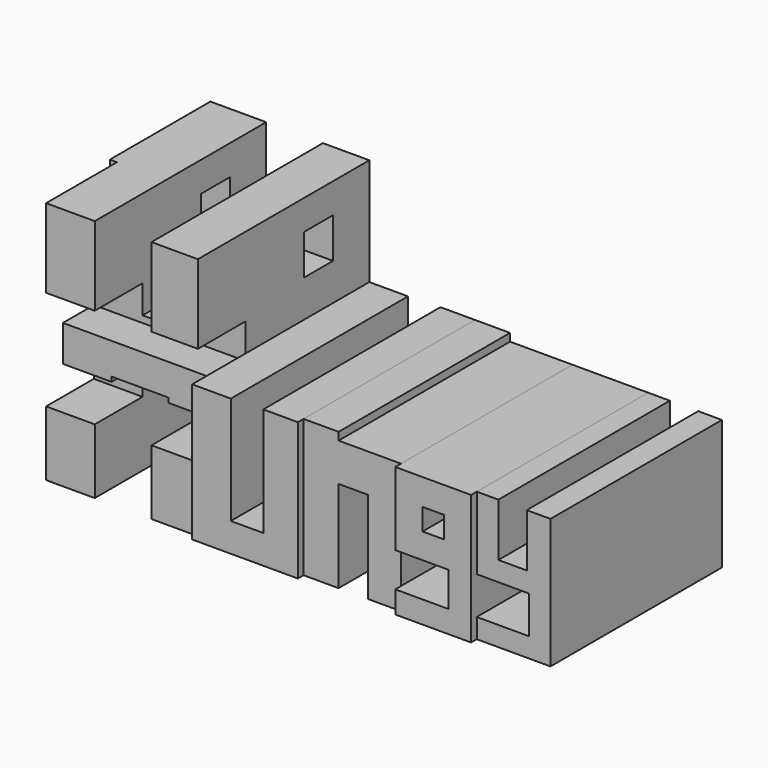
from build123d import *

# Parameters (mm, degrees)
F1_DEPTH = 76.2
F2_DEPTH = 78.74
F0_W     = 7.6985582709
F0_H     = 7.6985568739
F3_W     = 19.2463956773
F3_H     = 4.9490719102
F3_W_2   = 12.830927968
F3_H_2   = 14.2973195761
F3_H_3   = 10.814640671
F4_DEPTH = 179.3468610773
F5_DEPTH = 2.54


with BuildPart() as f1:
    # F0 (on Front) → F1 (new body)
    with BuildSketch(Plane.XZ):
        Polygon((-93.9285457134, 43.3502085507), (-93.9285457134, -43.3502085507), (-76.6189694405, -43.3502085507), (-76.6189694405, -8.3401026204), (-56.4560815692, -8.3401026204), (-56.4560815692, -43.3502085507), (-39.9591773748, -43.3502085507), (-39.9591773748, 5.224020686), (-39.9591773748, 43.3502085507), (-56.4560815692, 43.3502085507), (-56.4560815692, 5.224020686), (-76.6189694405, 5.224020686), (-76.6189694405, 43.3502085507), align=None)
    extrude(amount=F1_DEPTH)

    # F3 (on face) → F4 (cut, through all)
    with BuildSketch(Plane(origin=(-93.9285457134, 0, 0), x_dir=(0, -1, 0), z_dir=(-1, 0, 0))):
        with Locations((35.0886601955, -0.377497403)):
            Rectangle(F3_W, F3_H)
        Polygon((76.2, -20.2654339373), (76.2, 15.2945648879), (54.9766011536, 15.2945648879), (54.9766011536, 2.8302345891), (68.7240213156, 2.8302345891), (68.7240213156, -10.0006936118), (54.9766011536, -10.0006936118), (54.9766011536, -20.2654339373), align=None)
        with Locations((22.5326810032, 25.559307076)):
            Rectangle(F3_W_2, F3_H_2)
        with Locations((22.5326810032, -23.1065694243)):
            Rectangle(F3_W_2, F3_H_3)
    extrude(amount=-F4_DEPTH, mode=Mode.SUBTRACT)

    # F3 (on face) → F5 (join)
    with BuildSketch(Plane(origin=(-93.9285457134, 0, 0), x_dir=(0, -1, 0), z_dir=(-1, 0, 0))):
        Polygon((44.7118580341, 43.3502085507), (0, 43.3502085507), (0, -43.3502085507), (44.7118580341, -43.3502085507), (44.7118580341, -2.8520333581), (25.4654623568, -2.8520333581), (25.4654623568, 2.0970385522), (44.7118580341, 2.0970385522), align=None)
        with Locations((22.5326810032, -23.1065694243)):
            Rectangle(F3_W_2, F3_H_3, mode=Mode.SUBTRACT)
        with Locations((22.5326810032, 25.559307076)):
            Rectangle(F3_W_2, F3_H_2, mode=Mode.SUBTRACT)
    extrude(amount=F5_DEPTH)


with BuildPart() as f1b:
    # F0 (on Front) → F1, piece 2 (new body)
    with BuildSketch(Plane.XZ):
        Polygon((-2.3828870617, 5.590618588), (-2.3828870617, -43.3502085507), (10.081442073, -43.3502085507), (10.081442073, -10.7229892164), (20.529486239, -10.7229892164), (20.529486239, -43.3502085507), (32.2606191039, -43.3502085507), (32.2606191039, -35.4683510959), (32.2606191039, -23.1873188168), (32.2606191039, -10.7229892164), (32.2606191039, 2.8411338571), (10.081442073, 2.8411338571), (10.081442073, 5.590618588), align=None)
    extrude(amount=F1_DEPTH)


with BuildPart() as f1c:
    # F0 (on Front) → F1, piece 3 (new body)
    with BuildSketch(Plane.XZ):
        Polygon((66.9041201472, 2.8411338571), (59.2055656016, 2.8411338571), (59.2055656016, -23.0040214956), (77.7187645435, -23.0040214956), (77.7187645435, -36.3848470151), (59.2055656016, -36.3848470151), (59.2055656016, -43.3502085507), (77.7187645435, -43.3502085507), (85.4173153639, -43.3502085507), (85.4173153639, -23.0040214956), (85.4173153639, 2.8411338571), (76.9855678082, 2.8411338571), (76.9855678082, -16.03865996), (66.9041201472, -16.03865996), align=None)
    extrude(amount=F1_DEPTH)


with BuildPart() as f2:
    # F0 (on Front) → F2 (new body)
    with BuildSketch(Plane.XZ):
        Polygon((-39.9591773748, 5.224020686), (-39.9591773748, -43.3502085507), (-26.2117534876, -43.3502085507), (-14.6639179438, -43.3502085507), (-2.3828870617, -43.3502085507), (-2.3828870617, 5.590618588), (-14.6639179438, 5.590618588), (-14.6639179438, -33.0854654312), (-26.2117534876, -33.0854654312), (-26.2117534876, 5.224020686), align=None)
    extrude(amount=F2_DEPTH)


with BuildPart() as f2b:
    # F0 (on Front) → F2, piece 2 (new body)
    with BuildSketch(Plane.XZ):
        Polygon((59.2055656016, 2.8411338571), (32.2606191039, 2.8411338571), (32.2606191039, -10.7229892164), (32.2606191039, -23.1873188168), (51.1404126883, -23.1873188168), (51.1404126883, -35.4683510959), (32.2606191039, -35.4683510959), (32.2606191039, -43.3502085507), (51.1404126883, -43.3502085507), (59.2055656016, -43.3502085507), (59.2055656016, -36.3848470151), (59.2055656016, -23.1873188168), (59.2055656016, -23.0040214956), align=None)
        with Locations((45.8247438073, -10.3563915472)):
            Rectangle(F0_W, F0_H, mode=Mode.SUBTRACT)
    extrude(amount=F2_DEPTH)


solid = Compound([f1.part, f1b.part, f1c.part, f2.part, f2b.part])
